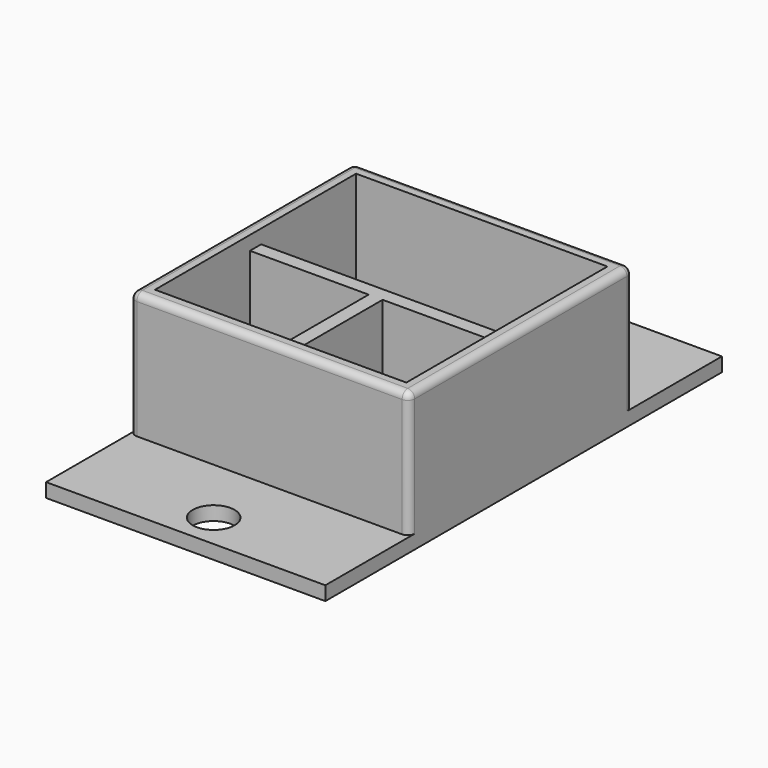
from build123d import *

# Parameters (mm, degrees)
F0_W     = 20
F0_H     = 20
F1_DEPTH = 10
F2_T     = -1
F4_DEPTH = 9
F5_W     = 20
F5_H     = 8
F5_R     = 1.5
F6_DEPTH = 1
F7_W     = 18
F7_H     = 18
F8_DEPTH = 1
F9_R     = 0.5


with BuildPart() as f1:
    # F0 (on Top) → F1 (new body)
    with BuildSketch(Plane.XY):
        Rectangle(F0_W, F0_H)
    extrude(amount=F1_DEPTH)

    # F2
    f2_openings = [f1.faces().sort_by_distance(p)[0] for p in [
        (0, 0, 0),
    ]]
    offset(amount=F2_T, openings=f2_openings)

    # F3 (on Top) → F4 (join)
    with BuildSketch(Plane.XY):
        Polygon((-0.5, -9), (0.5, -9), (0.5, -0.5), (9, -0.5), (9, 0.5), (0.5, 0.5), (-0.5, 0.5), (-9, 0.5), (-9, -0.5), (-0.5, -0.5), align=None)
    extrude(amount=F4_DEPTH)

    # F5 (on Top) → F6 (join)
    with BuildSketch(Plane.XY):
        with Locations((0, -13.5)):
            Rectangle(F5_W, F5_H)
        with Locations((0, -15)):
            Circle(F5_R, mode=Mode.SUBTRACT)
        with Locations((0, 14)):
            Rectangle(F5_W, F5_H)
        with Locations((0, 15)):
            Circle(F5_R, mode=Mode.SUBTRACT)
    extrude(amount=F6_DEPTH)

    # F7 (on face) → F8 (cut)
    with BuildSketch(Plane.XY.offset(10)):
        Rectangle(F7_W, F7_H)
    extrude(amount=-F8_DEPTH, mode=Mode.SUBTRACT)

    # F9
    f9_edges = [f1.edges().sort_by_distance(p)[0] for p in [
        (10, 0, 10),
        (0, -10, 10),
        (10, -10, 5.5),
        (-10, -10, 5.5),
        (10, 10, 5.5),
        (-10, 10, 5.5),
        (0, 10, 10),
        (-10, 0, 10),
    ]]
    fillet(f9_edges, radius=F9_R)


solid = f1.part
